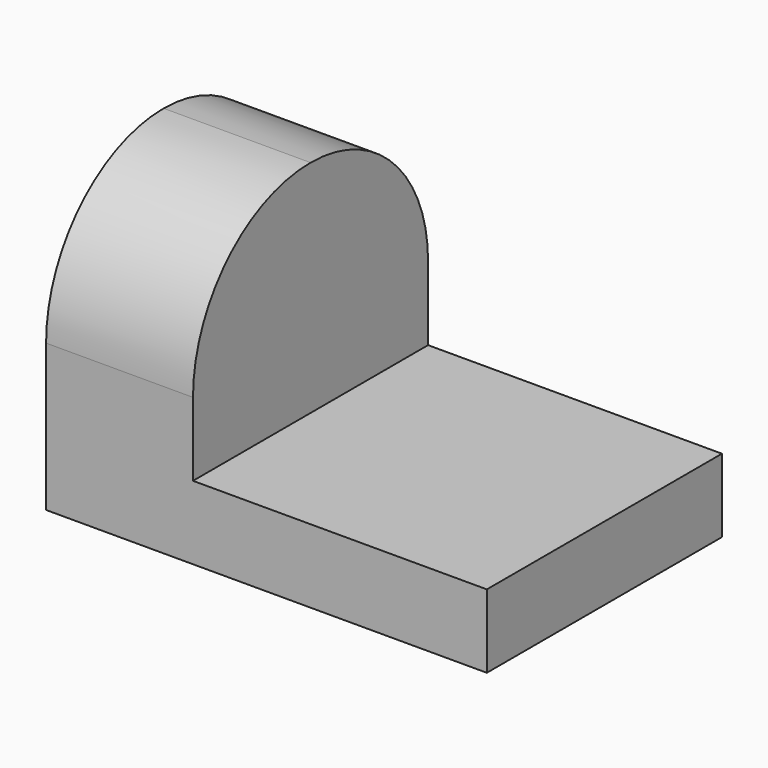
from build123d import *

# Parameters (mm, degrees)
F1_DEPTH = 12.7
F2_R     = 12.7
F3_R     = 12.69999


# Not quite as in the source:
# - a fillet or chamfer is up to 0.001 mm smaller than in the source, because OpenCascade refuses the exact size


with BuildPart() as f1:
    # F0 (on Front) → F1 (new body, symmetric)
    with BuildSketch(Plane.XZ):
        Polygon((0, 25.4), (0, 0), (38.1, 0), (38.1, 6.35), (12.7, 6.35), (12.7, 25.4), align=None)
    extrude(amount=F1_DEPTH, both=True)

    # F2
    f2_edges = [f1.edges().sort_by_distance(p)[0] for p in [
        (6.35, -12.7, 25.4),
    ]]
    fillet(f2_edges, radius=F2_R)

    # F3 (radius 12.7 in the source; OpenCascade refuses exactly that, so slightly less here)
    f3_edges = [f1.edges().sort_by_distance(p)[0] for p in [
        (6.35, 12.7, 25.4),
    ]]
    fillet(f3_edges, radius=F3_R)


solid = f1.part
